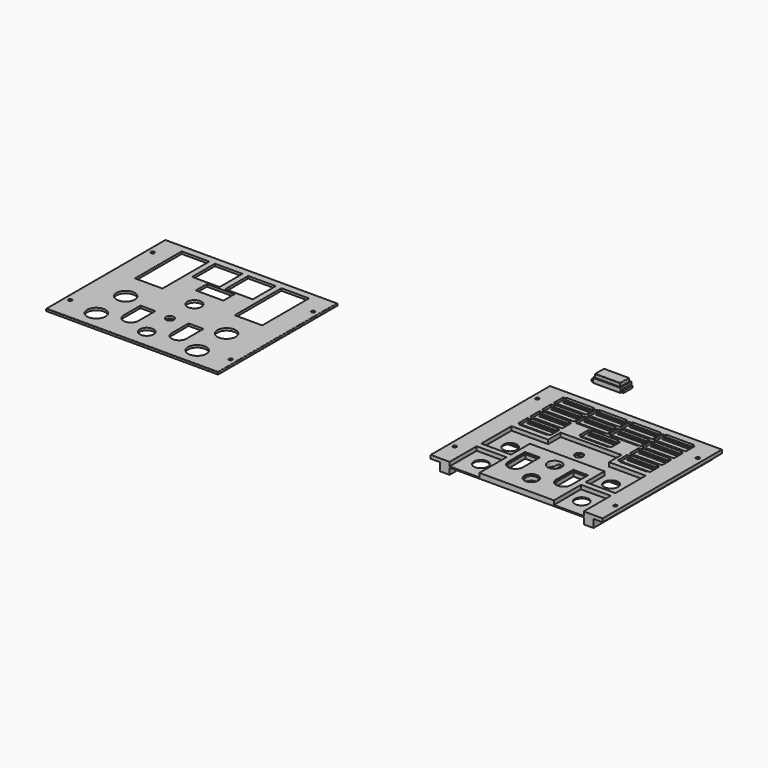
from build123d import *

# Parameters (mm, degrees)
F0_W      = 150
F0_H      = 130
F0_R      = 6.1
F0_R_2    = 1.5
F0_R_3    = 6
F1_DEPTH  = 10
F2_W      = 150
F2_H      = 130
F2_R      = 8
F2_R_2    = 1.5
F2_R_3    = 6
F2_R_4    = 3.5
F2_R_5    = 6.15
F2_W_2    = 5
F2_H_2    = 25
F3_DEPTH  = 2
F4_W      = 8
F4_H      = 7
F5_DEPTH  = 137.4
F6_R      = 6.1
F6_R_2    = 3.5
F7_DEPTH  = 3.5
F8_W      = 2
F8_H      = 10
F9_DEPTH  = 2
F10_W     = 18
F10_H     = 1
F10_H_2   = 17
F10_R     = 3.5
F11_DEPTH = 5.5
F12_R     = 6
F12_R_2   = 5
F13_DEPTH = 3.5
F14_W     = 29.5
F14_H     = 5
F15_DEPTH = 3.5
F17_W     = 1.9
F17_H     = 9.8
F18_DEPTH = 1.9
F19_W     = 24
F19_H     = 12
F20_DEPTH = 2
F21_W     = 22
F21_H     = 10
F22_DEPTH = 3
F23_W     = 22
F23_H     = 10
F24_DEPTH = 3
F16_W     = 24
F16_H     = 2
F25_DEPTH = 15
F27_DEPTH = 6
F29_DEPTH = 2
F30_R     = 0.5
F30_2_R   = 0.5


# Not quite as in the source:
# - a feature names something its author has since deleted; it is built from what else it names


with BuildPart() as f1:
    # F0 (on Top) → F1 (new body)
    with BuildSketch(Plane.XY):
        Rectangle(F0_W, F0_H)
        with Locations((-44, -49)):
            Circle(F0_R, mode=Mode.SUBTRACT)
        with Locations((-70, -45)):
            Circle(F0_R_2, mode=Mode.SUBTRACT)
        with BuildLine():
            Line((-27.5, -40), (-27.5, -21.5))
            Line((-27.5, -21.5), (-14.5, -21.5))
            Line((-14.5, -21.5), (-14.5, -40))
            ThreePointArc((-14.5, -40), (-16.4038059223, -44.5961940777), (-21, -46.5))
            ThreePointArc((-21, -46.5), (-25.5961940777, -44.5961940777), (-27.5, -40))
        make_face(mode=Mode.SUBTRACT)
        with Locations((-44, -17)):
            Circle(F0_R, mode=Mode.SUBTRACT)
        with Locations((0, -49)):
            Circle(F0_R_3, mode=Mode.SUBTRACT)
        with BuildLine():
            Line((14.5, -40), (14.5, -21.5))
            Line((14.5, -21.5), (27.5, -21.5))
            Line((27.5, -21.5), (27.5, -40))
            ThreePointArc((27.5, -40), (25.5961940777, -44.5961940777), (21, -46.5))
            ThreePointArc((21, -46.5), (16.4038059223, -44.5961940777), (14.5, -40))
        make_face(mode=Mode.SUBTRACT)
        with Locations((44, -49)):
            Circle(F0_R, mode=Mode.SUBTRACT)
        with Locations((70, -45)):
            Circle(F0_R_2, mode=Mode.SUBTRACT)
        with Locations((0, -23.6701526344)):
            Circle(F0_R_3, mode=Mode.SUBTRACT)
        with Locations((44, -17)):
            Circle(F0_R, mode=Mode.SUBTRACT)
        with Locations((-70, 45)):
            Circle(F0_R_2, mode=Mode.SUBTRACT)
        with BuildLine():
            ThreePointArc((0, 6.5), (2.4748737342, 5.4748737342), (3.5, 3))
            ThreePointArc((3.5, 3), (-2.4748737342, 0.5251262658), (0, 6.5))
        make_face(mode=Mode.SUBTRACT)
        with Locations((70, 45)):
            Circle(F0_R_2, mode=Mode.SUBTRACT)
    extrude(amount=F1_DEPTH)

    # F4 (on face) → F5 (cut)
    with BuildSketch(Plane.XZ.offset(65)):
        with Locations((-71, 3.5)):
            Rectangle(F4_W, F4_H)
        with Locations((71, 3.5)):
            Rectangle(F4_W, F4_H)
    extrude(amount=-F5_DEPTH, mode=Mode.SUBTRACT)

    # F6 (on face) → F7 (cut)
    with BuildSketch(Plane.XY.offset(10)):
        Polygon((-58.5, 2.5), (-58.5, -65), (-32.5, -65), (-32.5, -10), (32.5, -10), (32.5, -65), (58.5, -65), (58.5, 2.5), (26.5, 2.5), (26.5, 16), (17, 16), (-17, 16), (-26.5, 16), (-26.5, 2.5), align=None)
        with Locations((-44, -49)):
            Circle(F6_R, mode=Mode.SUBTRACT)
        with Locations((-44, -17)):
            Circle(F6_R, mode=Mode.SUBTRACT)
        with Locations((44, -49)):
            Circle(F6_R, mode=Mode.SUBTRACT)
        with Locations((44, -17)):
            Circle(F6_R, mode=Mode.SUBTRACT)
        with Locations((0, 3)):
            Circle(F6_R_2, mode=Mode.SUBTRACT)
    extrude(amount=-F7_DEPTH, mode=Mode.SUBTRACT)

    # F8 (on face) → F9 (cut)
    with BuildSketch(Plane.XY.offset(10)):
        Polygon((-55.5, 46.5), (-31.5, 46.5), (-31.5, 47.5), (-31.5, 57.5), (-31.5, 58.5), (-55.5, 58.5), (-55.5, 57.5), (-55.5, 47.5), align=None)
        with Locations((-30.5, 52.5)):
            Rectangle(F8_W, F8_H)
        with Locations((-56.5, 52.5)):
            Rectangle(F8_W, F8_H)
        Polygon((-31.5, 44.5), (-31.5, 45.5), (-55.5, 45.5), (-55.5, 44.5), (-55.5, 34.5), (-55.5, 33.5), (-31.5, 33.5), (-31.5, 34.5), align=None)
        with Locations((-30.5, 39.5)):
            Rectangle(F8_W, F8_H)
        with Locations((-56.5, 39.5)):
            Rectangle(F8_W, F8_H)
        Polygon((-31.5, 31.5), (-31.5, 32.5), (-55.5, 32.5), (-55.5, 31.5), (-55.5, 21.5), (-55.5, 20.5), (-31.5, 20.5), (-31.5, 21.5), align=None)
        with Locations((-30.5, 26.5)):
            Rectangle(F8_W, F8_H)
        with Locations((-56.5, 26.5)):
            Rectangle(F8_W, F8_H)
        Polygon((-31.5, 18.5), (-31.5, 19.5), (-55.5, 19.5), (-55.5, 18.5), (-55.5, 8.5), (-55.5, 7.5), (-31.5, 7.5), (-31.5, 8.5), align=None)
        with Locations((-30.5, 13.5)):
            Rectangle(F8_W, F8_H)
        with Locations((-56.5, 13.5)):
            Rectangle(F8_W, F8_H)
        with Locations((-27.5, 39.5)):
            Rectangle(F8_W, F8_H)
        Polygon((-26.5, 45.5), (-26.5, 44.5), (-26.5, 34.5), (-26.5, 33.5), (-2.5, 33.5), (-2.5, 34.5), (-2.5, 44.5), (-2.5, 45.5), align=None)
        with Locations((-1.5, 39.5)):
            Rectangle(F8_W, F8_H)
        Polygon((-26.5, 58.5), (-26.5, 57.5), (-26.5, 47.5), (-26.5, 46.5), (-2.5, 46.5), (-2.5, 47.5), (-2.5, 57.5), (-2.5, 58.5), align=None)
        with Locations((-27.5, 52.5)):
            Rectangle(F8_W, F8_H)
        with Locations((-1.5, 52.5)):
            Rectangle(F8_W, F8_H)
        with Locations((1.5, 39.5)):
            Rectangle(F8_W, F8_H)
        Polygon((2.5, 45.5), (2.5, 44.5), (2.5, 34.5), (2.5, 33.5), (26.5, 33.5), (26.5, 34.5), (26.5, 44.5), (26.5, 45.5), align=None)
        with Locations((27.5, 39.5)):
            Rectangle(F8_W, F8_H)
        Polygon((2.5, 58.5), (2.5, 57.5), (2.5, 47.5), (2.5, 46.5), (26.5, 46.5), (26.5, 47.5), (26.5, 57.5), (26.5, 58.5), align=None)
        with Locations((1.5, 52.5)):
            Rectangle(F8_W, F8_H)
        with Locations((27.5, 52.5)):
            Rectangle(F8_W, F8_H)
        with Locations((30.5, 39.5)):
            Rectangle(F8_W, F8_H)
        Polygon((31.5, 45.5), (31.5, 44.5), (31.5, 34.5), (31.5, 33.5), (55.5, 33.5), (55.5, 34.5), (55.5, 44.5), (55.5, 45.5), align=None)
        with Locations((56.5, 39.5)):
            Rectangle(F8_W, F8_H)
        Polygon((55.5, 19.5), (31.5, 19.5), (31.5, 18.5), (31.5, 8.5), (31.5, 7.5), (55.5, 7.5), (55.5, 8.5), (55.5, 18.5), align=None)
        with Locations((30.5, 13.5)):
            Rectangle(F8_W, F8_H)
        with Locations((56.5, 13.5)):
            Rectangle(F8_W, F8_H)
        Polygon((31.5, 20.5), (55.5, 20.5), (55.5, 21.5), (55.5, 31.5), (55.5, 32.5), (31.5, 32.5), (31.5, 31.5), (31.5, 21.5), align=None)
        with Locations((56.5, 26.5)):
            Rectangle(F8_W, F8_H)
        with Locations((30.5, 26.5)):
            Rectangle(F8_W, F8_H)
        Polygon((31.5, 58.5), (31.5, 57.5), (31.5, 47.5), (31.5, 46.5), (55.5, 46.5), (55.5, 47.5), (55.5, 57.5), (55.5, 58.5), align=None)
        with Locations((30.5, 52.5)):
            Rectangle(F8_W, F8_H)
        with Locations((56.5, 52.5)):
            Rectangle(F8_W, F8_H)
        Polygon((-12, 19.5), (12, 19.5), (12, 20.5), (12, 30.5), (12, 31.5), (-12, 31.5), (-12, 30.5), (-12, 20.5), align=None)
        with Locations((13, 25.5)):
            Rectangle(F8_W, F8_H)
        with Locations((-13, 25.5)):
            Rectangle(F8_W, F8_H)
    extrude(amount=-F9_DEPTH, mode=Mode.SUBTRACT)

    # F10 (on face) → F11 (cut)
    with BuildSketch(Plane.XY):
        Polygon((58.5, -65), (58.5, -5), (9, -5), (9, -6), (-9, -6), (-9, -5), (-58.5, -5), (-58.5, -65), align=None)
        with Locations((0, -5.5)):
            Rectangle(F10_W, F10_H)
        with Locations((0, 3.5)):
            Rectangle(F10_W, F10_H_2)
        with Locations((0, 3)):
            Circle(F10_R, mode=Mode.SUBTRACT)
    extrude(amount=F11_DEPTH, mode=Mode.SUBTRACT)

    # F12 (on face) → F13 (join)
    with BuildSketch(Plane(origin=(0, 0, 5.5), x_dir=(1, 0, 0), z_dir=(0, 0, -1))):
        with BuildLine():
            Line((-27.5, 40), (-27.5, 21.5))
            Line((-27.5, 21.5), (-14.5, 21.5))
            Line((-14.5, 21.5), (-14.5, 40))
            ThreePointArc((-14.5, 40), (-21, 46.5), (-27.5, 40))
        make_face()
        with BuildLine():
            ThreePointArc((-26.5, 40), (-21, 45.5), (-15.5, 40))
            Line((-15.5, 40), (-15.5, 22.5))
            Line((-15.5, 22.5), (-26.5, 22.5))
            Line((-26.5, 22.5), (-26.5, 40))
        make_face(mode=Mode.SUBTRACT)
        with BuildLine():
            Line((14.5, 40), (14.5, 21.5))
            Line((14.5, 21.5), (27.5, 21.5))
            Line((27.5, 21.5), (27.5, 40))
            ThreePointArc((27.5, 40), (21, 46.5), (14.5, 40))
        make_face()
        with BuildLine():
            ThreePointArc((15.5, 40), (21, 45.5), (26.5, 40))
            Line((26.5, 40), (26.5, 22.5))
            Line((26.5, 22.5), (15.5, 22.5))
            Line((15.5, 22.5), (15.5, 40))
        make_face(mode=Mode.SUBTRACT)
        with Locations((0, 49)):
            Circle(F12_R)
        with Locations((0, 49)):
            Circle(F12_R_2, mode=Mode.SUBTRACT)
    extrude(amount=-F13_DEPTH)

    # F14 (on face) → F15 (join)
    with BuildSketch(Plane.XY.offset(6.5)):
        with Locations((-47.25, -33)):
            Rectangle(F14_W, F14_H)
        with Locations((47.25, -33)):
            Rectangle(F14_W, F14_H)
    extrude(amount=F15_DEPTH)

    # F16 (on face) → F25 (cut)
    with BuildSketch(Plane.XY.offset(10)):
        with Locations((-43.5, 55.5)):
            Rectangle(F16_W, F16_H)
        with Locations((-43.5, 49.5)):
            Rectangle(F16_W, F16_H)
        with Locations((-43.5, 42.5)):
            Rectangle(F16_W, F16_H)
        with Locations((-43.5, 36.5)):
            Rectangle(F16_W, F16_H)
        with Locations((-43.5, 29.5)):
            Rectangle(F16_W, F16_H)
        with Locations((-43.5, 23.5)):
            Rectangle(F16_W, F16_H)
        with Locations((-43.5, 16.5)):
            Rectangle(F16_W, F16_H)
        with Locations((-43.5, 10.5)):
            Rectangle(F16_W, F16_H)
        with Locations((-14.5, 42.5)):
            Rectangle(F16_W, F16_H)
        with Locations((-14.5, 49.5)):
            Rectangle(F16_W, F16_H)
        with Locations((-14.5, 36.5)):
            Rectangle(F16_W, F16_H)
        with Locations((-14.5, 55.5)):
            Rectangle(F16_W, F16_H)
        with Locations((14.5, 42.5)):
            Rectangle(F16_W, F16_H)
        with Locations((14.5, 49.5)):
            Rectangle(F16_W, F16_H)
        with Locations((14.5, 36.5)):
            Rectangle(F16_W, F16_H)
        with Locations((14.5, 55.5)):
            Rectangle(F16_W, F16_H)
        with Locations((43.5, 42.5)):
            Rectangle(F16_W, F16_H)
        with Locations((43.5, 49.5)):
            Rectangle(F16_W, F16_H)
        with Locations((43.5, 29.5)):
            Rectangle(F16_W, F16_H)
        with Locations((43.5, 36.5)):
            Rectangle(F16_W, F16_H)
        with Locations((43.5, 16.5)):
            Rectangle(F16_W, F16_H)
        with Locations((43.5, 55.5)):
            Rectangle(F16_W, F16_H)
        with Locations((43.5, 10.5)):
            Rectangle(F16_W, F16_H)
        with Locations((43.5, 23.5)):
            Rectangle(F16_W, F16_H)
        with Locations((0, 28.5)):
            Rectangle(F16_W, F16_H)
        with Locations((0, 22.5)):
            Rectangle(F16_W, F16_H)
    extrude(amount=-F25_DEPTH, mode=Mode.SUBTRACT)

    # F26 (on face) → F27 (cut)
    with BuildSketch(Plane.XY):
        Polygon((60, 2.5), (60, 61), (-60, 61), (-60, 2.5), (-26.5, 2.5), (-26.5, 16), (26.5, 16), (26.5, 2.5), align=None)
    extrude(amount=F27_DEPTH, mode=Mode.SUBTRACT)

    # F28 (on face) → F29 (join)
    with BuildSketch(Plane(origin=(0, 0, 5.5), x_dir=(1, 0, 0), z_dir=(0, 0, -1))):
        with BuildLine():
            ThreePointArc((-1.5, 17.8606776151), (-0.7560257549, 17.7179744568), (0, 17.6701526344))
            ThreePointArc((0, 17.6701526344), (0.7560257549, 17.7179744568), (1.5, 17.8606776151))
            Line((1.5, 17.8606776151), (1.5, 29.4796276537))
            ThreePointArc((1.5, 29.4796276537), (0.7560257549, 29.622330812), (0, 29.6701526344))
            ThreePointArc((0, 29.6701526344), (-0.7560257549, 29.622330812), (-1.5, 29.4796276537))
            Line((-1.5, 29.4796276537), (-1.5, 17.8606776151))
        make_face()
        with BuildLine():
            ThreePointArc((0, 29.6701526344), (0.7560257549, 29.622330812), (1.5, 29.4796276537))
            Line((1.5, 29.4796276537), (1.5, 29.6701526344))
            Line((1.5, 29.6701526344), (0, 29.6701526344))
        make_face()
    extrude(amount=-F29_DEPTH)


with BuildPart() as f3:
    # F2 (on Top) → F3 (new body)
    with BuildSketch(Plane.XY):
        with Locations((-348.987051487, 16.9394645957)):
            Rectangle(F2_W, F2_H)
        with Locations((-392.987051487, -32.0605354043)):
            Circle(F2_R, mode=Mode.SUBTRACT)
        with Locations((-418.987051487, -28.0605354043)):
            Circle(F2_R_2, mode=Mode.SUBTRACT)
        with BuildLine():
            Line((-376.487051487, -23.0605354043), (-376.487051487, -4.5605354043))
            Line((-376.487051487, -4.5605354043), (-363.487051487, -4.5605354043))
            Line((-363.487051487, -4.5605354043), (-363.487051487, -23.0605354043))
            ThreePointArc((-363.487051487, -23.0605354043), (-365.3908574093, -27.656729482), (-369.987051487, -29.5605354043))
            ThreePointArc((-369.987051487, -29.5605354043), (-374.5832455647, -27.656729482), (-376.487051487, -23.0605354043))
        make_face(mode=Mode.SUBTRACT)
        with Locations((-392.987051487, -0.0605354043)):
            Circle(F2_R, mode=Mode.SUBTRACT)
        with Locations((-348.987051487, -32.0605354043)):
            Circle(F2_R_3, mode=Mode.SUBTRACT)
        with BuildLine():
            Line((-334.487051487, -23.0605354043), (-334.487051487, -4.5605354043))
            Line((-334.487051487, -4.5605354043), (-321.487051487, -4.5605354043))
            Line((-321.487051487, -4.5605354043), (-321.487051487, -23.0605354043))
            ThreePointArc((-321.487051487, -23.0605354043), (-323.3908574093, -27.656729482), (-327.987051487, -29.5605354043))
            ThreePointArc((-327.987051487, -29.5605354043), (-332.5832455647, -27.656729482), (-334.487051487, -23.0605354043))
        make_face(mode=Mode.SUBTRACT)
        with Locations((-304.987051487, -32.0605354043)):
            Circle(F2_R, mode=Mode.SUBTRACT)
        with Locations((-278.987051487, -28.0605354043)):
            Circle(F2_R_2, mode=Mode.SUBTRACT)
        with Locations((-348.987051487, -6.7305354043)):
            Circle(F2_R_4, mode=Mode.SUBTRACT)
        with Locations((-304.987051487, -0.0605354043)):
            Circle(F2_R, mode=Mode.SUBTRACT)
        with Locations((-418.987051487, 61.9394645957)):
            Circle(F2_R_2, mode=Mode.SUBTRACT)
        with Locations((-348.987051487, 19.9394645957)):
            Circle(F2_R_5, mode=Mode.SUBTRACT)
        Polygon((-404.487051487, 24.4394645957), (-404.487051487, 75.4394645957), (-380.487051487, 75.4394645957), (-375.487051487, 75.4394645957), (-351.487051487, 75.4394645957), (-346.487051487, 75.4394645957), (-322.487051487, 75.4394645957), (-317.487051487, 75.4394645957), (-293.487051487, 75.4394645957), (-293.487051487, 24.4394645957), (-317.487051487, 24.4394645957), (-317.487051487, 50.4394645957), (-322.487051487, 50.4394645957), (-336.987051487, 50.4394645957), (-336.987051487, 48.4394645957), (-336.987051487, 36.4394645957), (-360.987051487, 36.4394645957), (-360.987051487, 48.4394645957), (-360.987051487, 50.4394645957), (-375.487051487, 50.4394645957), (-380.487051487, 50.4394645957), (-380.487051487, 24.4394645957), align=None, mode=Mode.SUBTRACT)
        with Locations((-278.987051487, 61.9394645957)):
            Circle(F2_R_2, mode=Mode.SUBTRACT)
        with Locations((-377.987051487, 62.9394645957)):
            Rectangle(F2_W_2, F2_H_2)
        Polygon((-346.487051487, 75.4394645957), (-351.487051487, 75.4394645957), (-351.487051487, 50.4394645957), (-360.987051487, 50.4394645957), (-360.987051487, 48.4394645957), (-336.987051487, 48.4394645957), (-336.987051487, 50.4394645957), (-346.487051487, 50.4394645957), align=None)
        with Locations((-319.987051487, 62.9394645957)):
            Rectangle(F2_W_2, F2_H_2)
    extrude(amount=F3_DEPTH)

    # F30
    f30_edges = [f3.edges().sort_by_distance(p)[0] for p in [
        (-423.987051, 16.939465, 2),
        (-348.987051, -48.060535, 2),
        (-273.987051, 16.939465, 2),
        (-348.987051, 81.939465, 2),
    ]]
    fillet(f30_edges, radius=F30_R)


with BuildPart() as f18:
    # F17 (on Top) → F18 (new body)
    with BuildSketch(Plane.XY):
        Polygon((-67.1841184497, 101.9308240147), (-43.1841184497, 101.9308240147), (-43.1841184497, 103.0308240147), (-43.1841184497, 112.8308240147), (-43.1841184497, 113.9308240147), (-67.1841184497, 113.9308240147), (-67.1841184497, 112.8308240147), (-67.1841184497, 103.0308240147), align=None)
        with Locations((-42.2341184497, 107.9308240147)):
            Rectangle(F17_W, F17_H)
        with Locations((-68.1341184497, 107.9308240147)):
            Rectangle(F17_W, F17_H)
    extrude(amount=F18_DEPTH)

    # F19 (on face) → F20 (join)
    with BuildSketch(Plane.XY.offset(1.9)):
        with Locations((-55.1841184497, 107.9308240147)):
            Rectangle(F19_W, F19_H)
    extrude(amount=F20_DEPTH)

    # F21 (on face) → F22 (join)
    with BuildSketch(Plane.XY.offset(3.9)):
        with Locations((-55.1841184497, 107.9308240147)):
            Rectangle(F21_W, F21_H)
    extrude(amount=F22_DEPTH)

    # F23 (on face) → F24 (cut)
    with BuildSketch(Plane(origin=(0, 0, 0), x_dir=(1, 0, 0), z_dir=(0, 0, -1))):
        with Locations((-55.1841184497, -107.9308240147)):
            Rectangle(F23_W, F23_H)
    extrude(amount=-F24_DEPTH, mode=Mode.SUBTRACT)

    # F30#2
    f30_2_edges = [f18.edges().sort_by_distance(p)[0] for p in [
        (-66.184118, 107.930824, 6.9),
        (-55.184118, 112.930824, 6.9),
        (-44.184118, 107.930824, 6.9),
        (-55.184118, 102.930824, 6.9),
    ]]
    fillet(f30_2_edges, radius=F30_2_R)


solid = Compound([f1.part, f3.part, f18.part])
